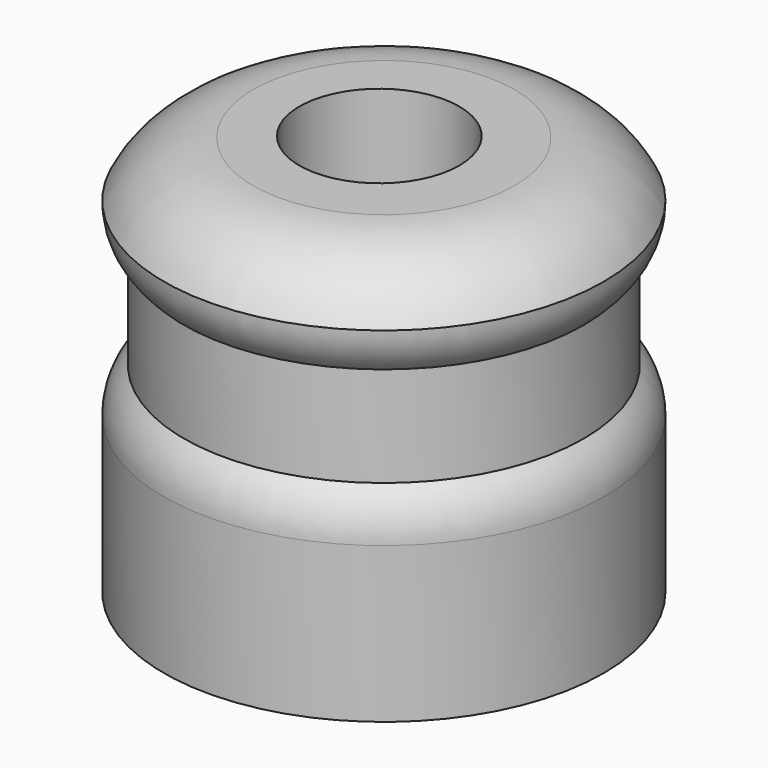
from build123d import *

# Parameters (mm, degrees)
F0_R     = 11
F0_R_2   = 4
F1_DEPTH = 10
F2_R     = 10
F2_R_2   = 4
F3_DEPTH = 5
F4_R     = 11
F4_R_2   = 10
F4_R_3   = 4
F5_DEPTH = 5


# Not quite as in the source:
# - a fillet or chamfer that OpenCascade refuses, or shapes differently, is made with other operations: its cross-section is extruded or revolved along the edge and cut away or added


with BuildPart() as f1:
    # F0 (on Top) → F1 (new body)
    with BuildSketch(Plane.XY):
        Circle(F0_R)
        with Locations((-0.2262097114, 0)):
            Circle(F0_R_2, mode=Mode.SUBTRACT)
    extrude(amount=F1_DEPTH)

    # F2 (on face) → F3 (join)
    with BuildSketch(Plane.XY.offset(10)):
        Circle(F2_R)
        with Locations((-0.2262097114, 0)):
            Circle(F2_R_2, mode=Mode.SUBTRACT)
    extrude(amount=F3_DEPTH)

    # F4 (on face) → F5 (join)
    with BuildSketch(Plane.XY.offset(15)):
        Circle(F4_R)
        Circle(F4_R_2, mode=Mode.SUBTRACT)
        Circle(F4_R_2)
        with Locations((-0.2262097114, 0)):
            Circle(F4_R_3, mode=Mode.SUBTRACT)
    extrude(amount=F5_DEPTH)

    # F6: fillet of radius 3 on 2 edges, made by hand

    # F6_s1 → F6_t2 (revolve, cut)
    with BuildSketch(Plane.XZ):
        with BuildLine():
            ThreePointArc((10, 15), (10.7386127875, 16.0113231061), (11, 17.2360679775))
            Line((11, 17.2360679775), (11, 15))
            Line((11, 15), (10, 15))
        make_face()
    revolve(axis=Axis((0, 0, 15), (0, 0, 1)), mode=Mode.SUBTRACT)

    # F6_s3 → F6_t4 (revolve, cut)
    with BuildSketch(Plane.XZ):
        with BuildLine():
            ThreePointArc((11, 7.7639320225), (10.7386127875, 8.9886768939), (10, 10))
            Line((10, 10), (11, 10))
            Line((11, 10), (11, 7.7639320225))
        make_face()
    revolve(axis=Axis((0, 0, 10), (0, 0, 1)), mode=Mode.SUBTRACT)

    # F7: fillet of radius 5 on 1 edges, made by hand

    # F7_s1 → F7_t2 (revolve, cut)
    with BuildSketch(Plane.XZ):
        with BuildLine():
            ThreePointArc((6.527864045, 20), (9.1565196056, 19.2532540418), (11, 17.2360679775))
            Line((11, 17.2360679775), (11, 20))
            Line((11, 20), (6.527864045, 20))
        make_face()
    revolve(axis=Axis((0, 0, 20), (0, 0, 1)), mode=Mode.SUBTRACT)


solid = f1.part
